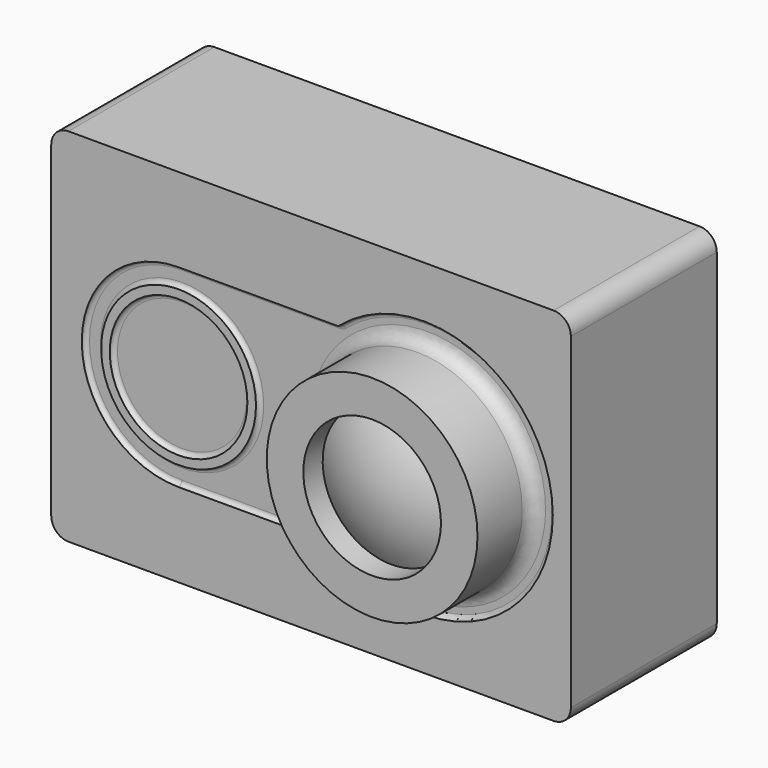
from build123d import *

# Parameters (mm, degrees)
F0_W     = 60.4
F0_H     = 42
F1_DEPTH = 21.2
F2_R     = 2
F3_R     = 9
F3_R_2   = 12.25
F4_DEPTH = 0.5
F3_R_3   = 8
F5_DEPTH = 0.5
F6_DEPTH = 7.5
F10_R    = 1.5
F11_R    = 0.49999
F12_R    = 0.49999


# Not quite as in the source:
# - a fillet or chamfer is up to 0.001 mm smaller than in the source, because OpenCascade refuses the exact size


with BuildPart() as f1:
    # F0 (on Front) → F1 (new body)
    with BuildSketch(Plane.XZ):
        with Locations((0, 21)):
            Rectangle(F0_W, F0_H)
    extrude(amount=F1_DEPTH)

    # F2
    f2_edges = [f1.edges().sort_by_distance(p)[0] for p in [
        (-30.2, -10.6, 42),
        (30.2, -10.6, 42),
        (30.2, -10.6, 0),
        (-30.2, -10.6, 0),
    ]]
    fillet(f2_edges, radius=F2_R)

    # F3 (on face) → F4 (cut)
    with BuildSketch(Plane.XZ.offset(21.2)):
        with BuildLine():
            ThreePointArc((2.9912166904, 9.75), (3.1651187763, 9.7187836009), (3.3173064746, 9.6290322581))
            ThreePointArc((3.3173064746, 9.6290322581), (28.1, 21), (3.3173064746, 32.3709677419))
            ThreePointArc((3.3173064746, 32.3709677419), (3.1651187763, 32.2812163991), (2.9912166904, 32.25))
            Line((2.9912166904, 32.25), (-15.4, 32.25))
            ThreePointArc((-15.4, 32.25), (-26.65, 21), (-15.4, 9.75))
            Line((-15.4, 9.75), (2.9912166904, 9.75))
        make_face()
        with Locations((-15.4, 21)):
            Circle(F3_R, mode=Mode.SUBTRACT)
        with Locations((13.1, 21)):
            Circle(F3_R_2, mode=Mode.SUBTRACT)
    extrude(amount=-F4_DEPTH, mode=Mode.SUBTRACT)

    # F3 (on face) → F5 (cut)
    with BuildSketch(Plane.XZ.offset(21.2)):
        with Locations((-15.4, 21)):
            Circle(F3_R_3)
    extrude(amount=-F5_DEPTH, mode=Mode.SUBTRACT)

    # F3 (on face) → F6 (join)
    with BuildSketch(Plane.XZ.offset(21.2)):
        with Locations((13.1, 21)):
            Circle(F3_R_2)
    extrude(amount=F6_DEPTH)

    # F8 (on offset) → F9 (revolve, cut)
    with BuildSketch(Plane.YZ.offset(13.1)):
        with BuildLine():
            ThreePointArc((-28.2, 21), (-27.6105631935, 25.1636124275), (-25.8885775404, 29))
            Line((-25.8885775404, 29), (-28.7, 29))
            Line((-28.7, 29), (-28.7, 21))
            Line((-28.7, 21), (-28.2, 21))
        make_face()
    revolve(axis=Axis((13.1, -14.35, 21), (0, 1, 0)), mode=Mode.SUBTRACT)

    # F10
    f10_edges = [f1.edges().sort_by_distance(p)[0] for p in [
        (0.85, -20.7, 21),
    ]]
    fillet(f10_edges, radius=F10_R)

    # F11 (radius 0.5 in the source; OpenCascade refuses exactly that, so slightly less here)
    f11_edges = [f1.edges().sort_by_distance(p)[0] for p in [
        (-0.65, -20.7, 21),
        (-6.204392, -20.7, 9.75),
        (3.165119, -20.7, 9.718784),
        (28.1, -20.7, 21),
        (3.165119, -20.7, 32.281216),
        (-6.204392, -20.7, 32.25),
        (-26.65, -20.7, 21),
        (-24.4, -20.7, 21),
    ]]
    fillet(f11_edges, radius=F11_R)

    # F12 (radius 0.5 in the source; OpenCascade refuses exactly that, so slightly less here)
    f12_edges = [f1.edges().sort_by_distance(p)[0] for p in [
        (-23.4, -20.7, 21),
    ]]
    fillet(f12_edges, radius=F12_R)


solid = f1.part
